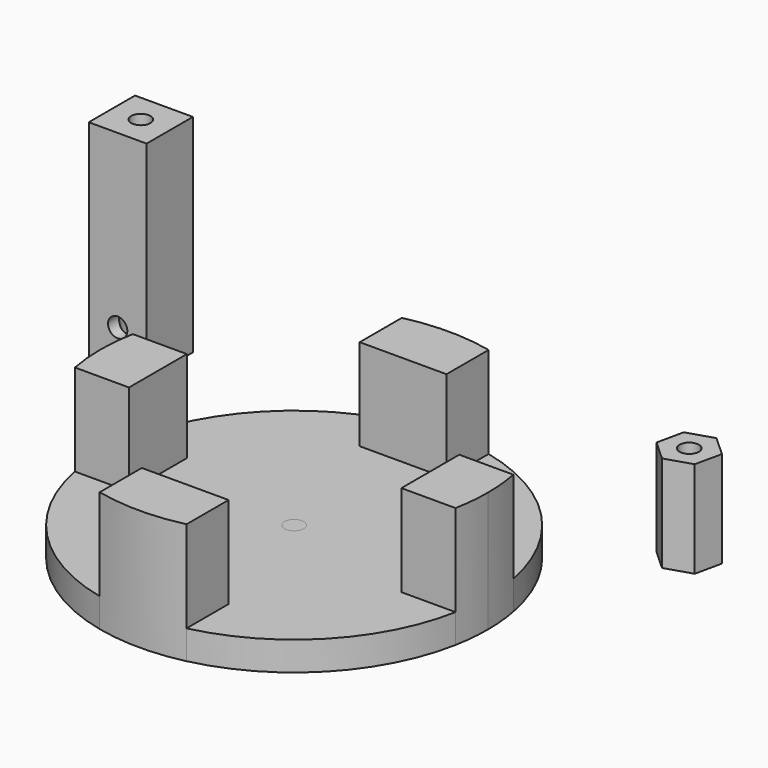
from build123d import *

# Parameters (mm, degrees)
F1_DEPTH  = 25
F2_DEPTH  = 6
F5_DEPTH  = 20
F6_R      = 2
F7_DEPTH  = 10
F3_R      = 2
F9_DEPTH  = 25
F10_W     = 14.5
F10_H     = 14.5
F11_DEPTH = 2
F12_W     = 12
F12_H     = 12
F13_DEPTH = 43
F14_R     = 2
F15_DEPTH = 14
F16_R     = 3.75
F17_DEPTH = 29
F18_R     = 2
F19_DEPTH = 20


with BuildPart() as f1:
    # F0 (on Top) → F1 (new body)
    with BuildSketch(Plane.XY):
        with BuildLine():
            Line((-28.25, 7.5), (-39.4705935011, 7.5))
            ThreePointArc((-39.4705935011, 7.5), (-40.1768310265, 0), (-39.4705935011, -7.5))
            Line((-39.4705935011, -7.5), (-28.25, -7.5))
            Line((-28.25, -7.5), (-28.25, 7.5))
        make_face()
    extrude(amount=F1_DEPTH)



with BuildPart() as f1b:
    # F0 (on Top) → F1, piece 2 (new body)
    with BuildSketch(Plane.XY):
        with BuildLine():
            Line((-9, 28.25), (9, 28.25))
            Line((9, 28.25), (9, 39.1558137616))
            ThreePointArc((9, 39.1558137616), (0, 40.1768310265), (-9, 39.1558137616))
            Line((-9, 39.1558137616), (-9, 28.25))
        make_face()
    extrude(amount=F1_DEPTH)


with BuildPart() as f1c:
    # F0 (on Top) → F1, piece 3 (new body)
    with BuildSketch(Plane.XY):
        with BuildLine():
            ThreePointArc((40.1768310265, 0), (39.9998819807, 3.766589022), (39.4705935011, 7.5))
            Line((39.4705935011, 7.5), (28.25, 7.5))
            Line((28.25, 7.5), (28.25, -7.5))
            Line((28.25, -7.5), (39.4705935011, -7.5))
            ThreePointArc((39.4705935011, -7.5), (39.9998819807, -3.766589022), (40.1768310265, 0))
        make_face()
    extrude(amount=F1_DEPTH)


with BuildPart() as f1d:
    # F0 (on Top) → F1, piece 4 (new body)
    with BuildSketch(Plane.XY):
        with BuildLine():
            Line((-9, -28.25), (-9, -39.1558137616))
            ThreePointArc((-9, -39.1558137616), (0, -40.1768310265), (9, -39.1558137616))
            Line((9, -39.1558137616), (9, -28.25))
            Line((9, -28.25), (-9, -28.25))
        make_face()
    extrude(amount=F1_DEPTH)


with BuildPart() as f1_1:
    add(f1.part)

    add(f1b.part)  # F2 merges F1b

    add(f1c.part)  # F2 merges F1c

    add(f1d.part)  # F2 merges F1d
    # F0 (on Top) → F2 (join)
    with BuildSketch(Plane.XY):
        with BuildLine():
            Line((9, 39.1558137616), (9, 28.25))
            Line((9, 28.25), (-9, 28.25))
            Line((-9, 28.25), (-9, 39.1558137616))
            ThreePointArc((-9, 39.1558137616), (-28.9460229533, 27.8622595372), (-39.4705935011, 7.5))
            Line((-39.4705935011, 7.5), (-28.25, 7.5))
            Line((-28.25, 7.5), (-28.25, -7.5))
            Line((-28.25, -7.5), (-39.4705935011, -7.5))
            ThreePointArc((-39.4705935011, -7.5), (-28.9460229533, -27.8622595372), (-9, -39.1558137616))
            Line((-9, -39.1558137616), (-9, -28.25))
            Line((-9, -28.25), (9, -28.25))
            Line((9, -28.25), (9, -39.1558137616))
            ThreePointArc((9, -39.1558137616), (28.9460229533, -27.8622595372), (39.4705935011, -7.5))
            Line((39.4705935011, -7.5), (28.25, -7.5))
            Line((28.25, -7.5), (28.25, 7.5))
            Line((28.25, 7.5), (39.4705935011, 7.5))
            ThreePointArc((39.4705935011, 7.5), (28.9460229533, 27.8622595372), (9, 39.1558137616))
        make_face()
    extrude(amount=F2_DEPTH)


with BuildPart() as f5:
    # F4 (on Top) → F5 (new body)
    with BuildSketch(Plane.XY):
        Polygon((48.7069180292, 34.488302664), (54.1130541824, 36.2042821944), (55.3300403933, 41.7441232045), (51.140890451, 45.5679846843), (45.7347542979, 43.8520051539), (44.517768087, 38.3121641438), align=None)
    extrude(amount=F5_DEPTH)

    # F6 (on face) → F7 (cut)
    with BuildSketch(Plane.XY.offset(20)):
        with Locations((49.9239042401, 40.0281436741)):
            Circle(F6_R)
    extrude(amount=-F7_DEPTH, mode=Mode.SUBTRACT)


with BuildPart() as f8_1:
    # F8: copy of F1
    add(f1_1.part)

    # F3 (on face) → F9 (cut)
    with BuildSketch(Plane(origin=(0, 0, 0), x_dir=(1, 0, 0), z_dir=(0, 0, -1))):
        Circle(F3_R)
    extrude(amount=-F9_DEPTH, mode=Mode.SUBTRACT)

    # F10 (on face) → F11 (cut)
    with BuildSketch(Plane(origin=(0, 0, 0), x_dir=(1, 0, 0), z_dir=(0, 0, -1))):
        Rectangle(F10_W, F10_H)
    extrude(amount=-F11_DEPTH, mode=Mode.SUBTRACT)


with BuildPart() as f13:
    # F12 (on Top) → F13 (new body)
    with BuildSketch(Plane.XY):
        with Locations((-63.8585659266, 40.0724475682)):
            Rectangle(F12_W, F12_H)
    extrude(amount=F13_DEPTH)

    # F14 (on face) → F15 (cut)
    with BuildSketch(Plane.XY.offset(43)):
        with Locations((-63.8585659266, 40.0724475682)):
            Circle(F14_R)
    extrude(amount=-F15_DEPTH, mode=Mode.SUBTRACT)

    # F16 (on face) → F17 (cut)
    with BuildSketch(Plane(origin=(0, 0, 0), x_dir=(1, 0, 0), z_dir=(0, 0, -1))):
        with Locations((-63.8585659266, -40.0724475682)):
            Circle(F16_R)
    extrude(amount=-F17_DEPTH, mode=Mode.SUBTRACT)

    # F18 (on face) → F19 (cut)
    with BuildSketch(Plane.XZ.offset(-34.0724475682)):
        with Locations((-63.8585659266, 7.5)):
            Circle(F18_R)
    extrude(amount=-F19_DEPTH, mode=Mode.SUBTRACT)


solid = Compound([f1_1.part, f5.part, f8_1.part, f13.part])
